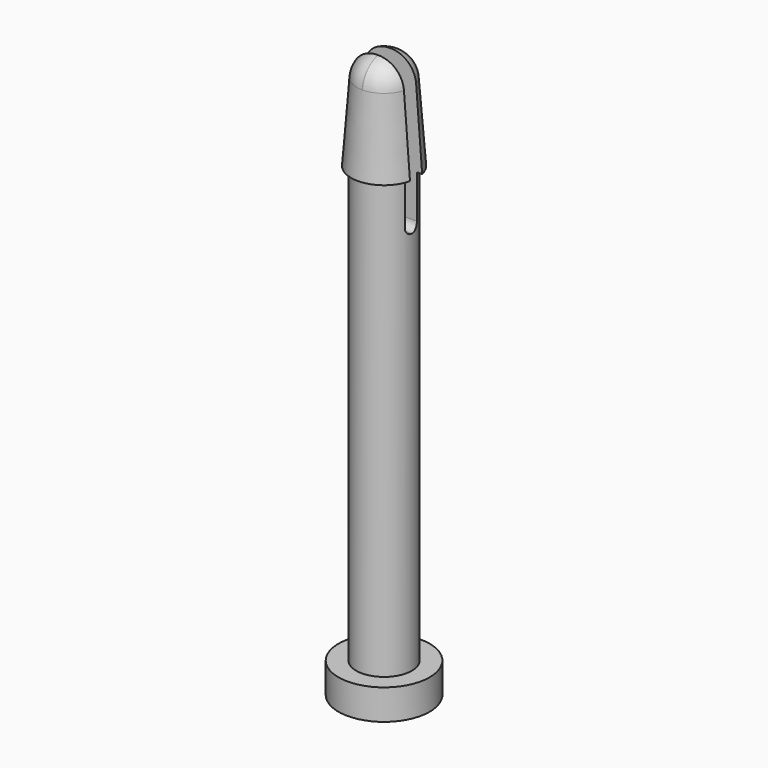
from build123d import *

# Parameters (mm, degrees)
F0_R        = 4.5
F1_DEPTH    = 3
F2_R        = 2.75
F3_DEPTH    = 43
F6_W        = 10
F6_H        = 1.5
F7_DEPTH    = 15
F8_T2_ANGLE = 359.64
F8_T4_ANGLE = 359.64
F9_R        = 0.7499


# Not quite as in the source:
# - a fillet or chamfer that OpenCascade refuses, or shapes differently, is made with other operations: its cross-section is extruded or revolved along the edge and cut away or added
# - a fillet or chamfer is up to 0.001 mm smaller than in the source, because OpenCascade refuses the exact size


with BuildPart() as f1:
    # F0 (on Top) → F1 (new body)
    with BuildSketch(Plane.XY):
        Circle(F0_R)
    extrude(amount=F1_DEPTH)

    # F2 (on face) → F3 (join)
    with BuildSketch(Plane.XY.offset(3)):
        Circle(F2_R)
    extrude(amount=F3_DEPTH)

    # F4 (on Front) → F5 (revolve)
    with BuildSketch(Plane.XZ):
        Polygon((0, 56), (0, 46), (3.25, 46), (2.5, 56), align=None)
    revolve(axis=Axis((0, 0, 51), (0, 0, -1)))

    # F6 (on face) → F7 (cut)
    with BuildSketch(Plane.XY.offset(56)):
        Rectangle(F6_W, F6_H)
    extrude(amount=-F7_DEPTH, mode=Mode.SUBTRACT)

    # F8: fillet of radius 2.5 on 2 edges, made by hand

    # F8_s1 → F8_t2 (revolve, cut)
    with BuildSketch(Plane(origin=(0, 0, 0), x_dir=(0, 0, 1), z_dir=(0.9999950652, -0.0031415875, 0))):
        with BuildLine():
            ThreePointArc((56, 0.18047861), (55.3326807109, 1.880855454), (53.6869748706, 2.6734768847))
            Line((53.6869748706, 2.6734768847), (56, 2.5))
            Line((56, 2.5), (56, 0.18047861))
        make_face()
    revolve(axis=Axis((0, 0, 56), (0, 0, -1)), revolution_arc=F8_T2_ANGLE, mode=Mode.SUBTRACT)

    # F8_s3 → F8_t4 (revolve, cut)
    with BuildSketch(Plane(origin=(0, 0, 0), x_dir=(0, 0, 1), z_dir=(-0.9999950652, 0.0031415875, 0))):
        with BuildLine():
            ThreePointArc((53.6869748706, 2.6734768847), (55.3326807109, 1.880855454), (56, 0.18047861))
            Line((56, 0.18047861), (56, 2.5))
            Line((56, 2.5), (53.6869748706, 2.6734768847))
        make_face()
    revolve(axis=Axis((0, 0, 56), (0, 0, -1)), revolution_arc=F8_T4_ANGLE, mode=Mode.SUBTRACT)

    # F9 (radius 0.75 in the source; OpenCascade refuses exactly that, so slightly less here)
    f9_edges = [f1.edges().sort_by_distance(p)[0] for p in [
        (0, 0.75, 41),
        (0, -0.75, 41),
    ]]
    fillet(f9_edges, radius=F9_R)


solid = f1.part
